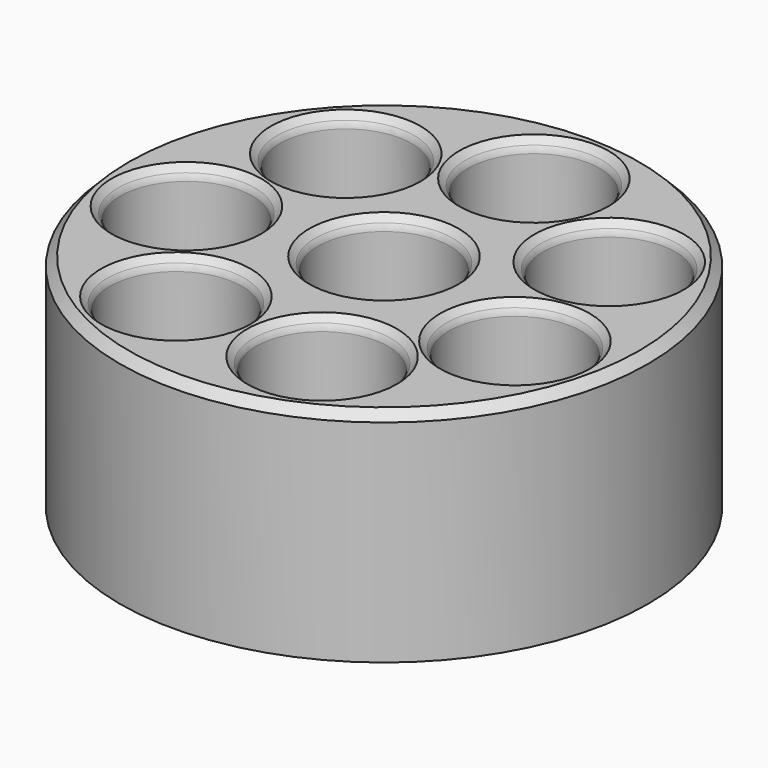
from build123d import *

# Parameters (mm, degrees)
F0_R     = 30
F0_R_2   = 7.5
F1_DEPTH = 25
F2_DEPTH = 2
F3_R     = 7.5
F3_R_2   = 2.9
F4_DEPTH = 1.5
F5_SIZE  = 1
F6_R     = 1


# Not quite as in the source:
# - a feature names something its author has since deleted; it is built from what else it names


with BuildPart() as f1:
    # F0 (on Top) → F1 (new body)
    with BuildSketch(Plane.XY):
        with Locations((14.9640348837, -13.26942576)):
            Circle(F0_R)
        with Locations((5.3571123497, -30.8110060601)):
            Circle(F0_R_2, mode=Mode.SUBTRACT)
        with Locations((-4.7403430744, -16.6954276989)):
            Circle(F0_R_2, mode=Mode.SUBTRACT)
        with Locations((22.6887763873, -31.7174166723)):
            Circle(F0_R_2, mode=Mode.SUBTRACT)
        with Locations((34.2035525167, -18.7321138571)):
            Circle(F0_R_2, mode=Mode.SUBTRACT)
        Circle(F0_R_2, mode=Mode.SUBTRACT)
        with Locations((14.9640348837, -13.26942576)):
            Circle(F0_R_2, mode=Mode.SUBTRACT)
        with Locations((31.2305794538, -1.6332954863)):
            Circle(F0_R_2, mode=Mode.SUBTRACT)
        with Locations((16.0085665525, 6.7032794547)):
            Circle(F0_R_2, mode=Mode.SUBTRACT)
    extrude(amount=F1_DEPTH)

    # F0 (on Top) → F2 (join)
    with BuildSketch(Plane.XY):
        with Locations((31.2305794538, -1.6332954863)):
            Circle(F0_R_2)
        with Locations((34.2035525167, -18.7321138571)):
            Circle(F0_R_2)
        with Locations((22.6887763873, -31.7174166723)):
            Circle(F0_R_2)
        with Locations((14.9640348837, -13.26942576)):
            Circle(F0_R_2)
        with Locations((16.0085665525, 6.7032794547)):
            Circle(F0_R_2)
        Circle(F0_R_2)
        with Locations((5.3571123497, -30.8110060601)):
            Circle(F0_R_2)
        with Locations((-4.7403430744, -16.6954276989)):
            Circle(F0_R_2)
    extrude(amount=F2_DEPTH)

    # F3 (on face) → F4 (join)
    with BuildSketch(Plane.XY.offset(2)):
        with Locations((5.3571123497, -30.8110060601)):
            Circle(F3_R)
        with Locations((5.3571123497, -30.8110060601)):
            Circle(F3_R_2, mode=Mode.SUBTRACT)
        with Locations((14.9640348837, -13.26942576)):
            Circle(F3_R)
        with Locations((14.9640348837, -13.26942576)):
            Circle(F3_R_2, mode=Mode.SUBTRACT)
        with Locations((22.6887763873, -31.7174166723)):
            Circle(F3_R)
        with Locations((22.6887763873, -31.7174166723)):
            Circle(F3_R_2, mode=Mode.SUBTRACT)
        with Locations((34.2035525167, -18.7321138571)):
            Circle(F3_R)
        with Locations((34.2035525167, -18.7321138571)):
            Circle(F3_R_2, mode=Mode.SUBTRACT)
        with Locations((31.2305794538, -1.6332954863)):
            Circle(F3_R)
        with Locations((31.2305794538, -1.6332954863)):
            Circle(F3_R_2, mode=Mode.SUBTRACT)
        with Locations((16.0085665525, 6.7032794547)):
            Circle(F3_R)
        with Locations((16.0085665525, 6.7032794547)):
            Circle(F3_R_2, mode=Mode.SUBTRACT)
        with Locations((-4.7403430744, -16.6954276989)):
            Circle(F3_R)
        with Locations((-4.7403430744, -16.6954276989)):
            Circle(F3_R_2, mode=Mode.SUBTRACT)
        Circle(F3_R)
        Circle(F3_R_2, mode=Mode.SUBTRACT)
    extrude(amount=F4_DEPTH)

    # F5
    f5_edges = [f1.edges().sort_by_distance(p)[0] for p in [
        (-12.240343, -16.695428, 25),
        (-7.5, 0, 25),
        (8.508567, 6.703279, 25),
        (23.730579, -1.633295, 25),
        (26.703553, -18.732114, 25),
        (7.464035, -13.269426, 25),
        (-2.142888, -30.811006, 25),
        (15.188776, -31.717417, 25),
        (-15.035965, -13.269426, 25),
    ]]
    chamfer(f5_edges, length=F5_SIZE)

    # F6
    f6_edges = [f1.edges().sort_by_distance(p)[0] for p in [
        (-2.142888, -30.811006, 24),
        (-12.240343, -16.695428, 24),
        (15.188776, -31.717417, 24),
        (26.703553, -18.732114, 24),
        (23.730579, -1.633295, 24),
        (8.508567, 6.703279, 24),
        (-7.5, 0, 24),
        (7.464035, -13.269426, 24),
        (2.457112, -30.811006, 2),
        (-7.640343, -16.695428, 2),
        (-2.9, 0, 3.5),
        (12.064035, -13.269426, 2),
        (19.788776, -31.717417, 3.5),
        (31.303553, -18.732114, 2),
        (28.330579, -1.633295, 3.5),
        (13.108567, 6.703279, 2),
        (8.508567, 6.703279, 3.5),
        (7.464035, -13.269426, 3.5),
        (-7.5, 0, 3.5),
        (-12.240343, -16.695428, 3.5),
        (-2.142888, -30.811006, 3.5),
        (15.188776, -31.717417, 3.5),
        (26.703553, -18.732114, 3.5),
        (23.730579, -1.633295, 3.5),
    ]]
    fillet(f6_edges, radius=F6_R)


solid = f1.part
